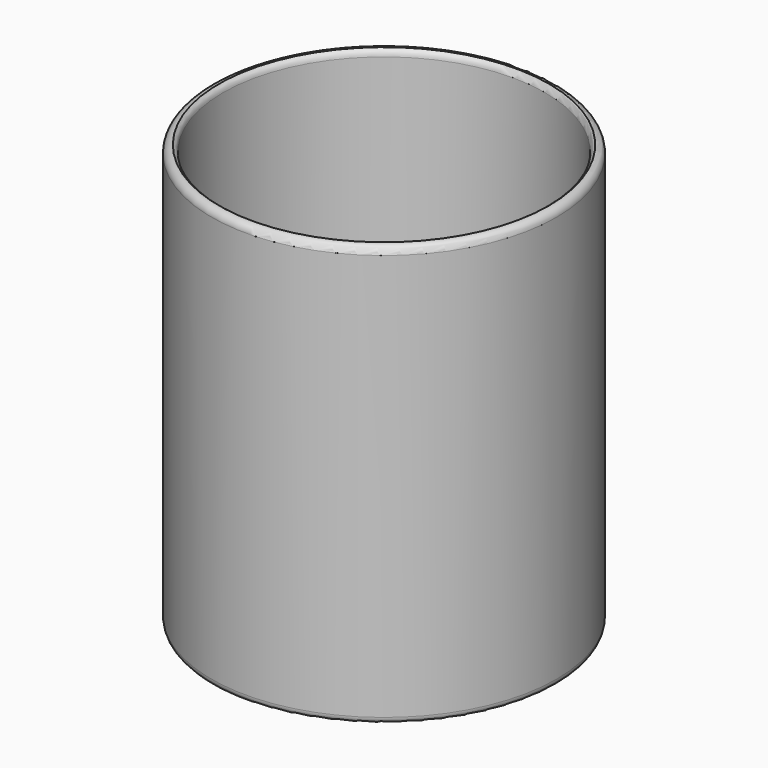
from build123d import *

# Parameters (mm, degrees)
F0_R     = 45
F1_DEPTH = 110
F2_T     = -3
F3_R     = 2
F4_R     = 2
F5_R     = 2
F7_DEPTH = 1


# Not quite as in the source:
# - a fillet or chamfer that OpenCascade refuses, or shapes differently, is made with other operations: its cross-section is extruded or revolved along the edge and cut away or added


with BuildPart() as f1:
    # F0 (on Top) → F1 (new body)
    with BuildSketch(Plane.XY):
        Circle(F0_R)
    extrude(amount=F1_DEPTH)

    # F2
    f2_openings = [f1.faces().sort_by_distance(p)[0] for p in [
        (0, 0, 110),
    ]]
    offset(amount=F2_T, openings=f2_openings)

    # F3
    f3_edges = [f1.edges().sort_by_distance(p)[0] for p in [
        (-42, 0, 3),
    ]]
    fillet(f3_edges, radius=F3_R)

    # F4
    f4_edges = [f1.edges().sort_by_distance(p)[0] for p in [
        (-45, 0, 0),
    ]]
    fillet(f4_edges, radius=F4_R)

    # F5
    f5_edges = [f1.edges().sort_by_distance(p)[0] for p in [
        (-45, 0, 110),
    ]]
    fillet(f5_edges, radius=F5_R)

    # F6: fillet of radius 2 on 1 edges, made by hand

    # F6_s1 → F6_t2 (revolve, cut)
    with BuildSketch(Plane.XZ):
        with BuildLine():
            ThreePointArc((42.9997999035, 110.0003463544), (42.2675927526, 109.2678330874), (41.9996, 108.2673917434))
            Line((41.9996, 108.2673917434), (41.7994634315, 108.2673917434))
            ThreePointArc((41.7994634315, 108.2673917434), (41.7998634315, 109.1336958717), (41.7998634315, 110))
            Line((41.7998634315, 110), (42, 110.2001365685))
            ThreePointArc((42, 110.2001365685), (42.4998999517, 110.2001365685), (42.8996833253, 110.1736418155))
            Line((42.8996833253, 110.1736418155), (42.9997999035, 110.0003463544))
        make_face()
    revolve(axis=Axis((0, 0, 110), (0, 0, 1)), mode=Mode.SUBTRACT)

    # F7 (cut): a face of the model
    f7_faces = [f1.faces().sort_by_distance(p)[0] for p in [
        (0, 0, 0),
    ]]
    extrude(f7_faces, amount=-F7_DEPTH, mode=Mode.SUBTRACT)

    # F8: fillet of radius 1 on 1 edges, made by hand

    # F8_s1 → F8_t2 (revolve, cut)
    with BuildSketch(Plane.XZ):
        with BuildLine():
            ThreePointArc((44.7320508076, 1), (43.8660254038, 0.5), (43, 1))
            Line((43, 1), (43, 0))
            ThreePointArc((43, 0), (44, 0.2679491924), (44.7320508076, 1))
        make_face()
    revolve(axis=Axis((0, 0, 0), (0, 0, 1)), mode=Mode.SUBTRACT)


solid = f1.part
